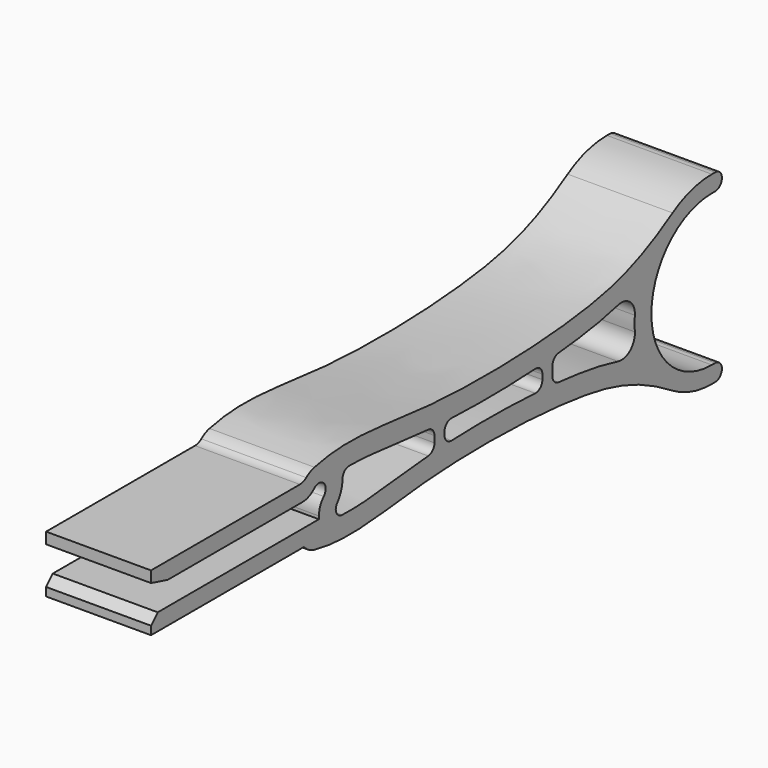
from build123d import *

# Parameters (mm, degrees)
F1_DEPTH    = 25
F2_T        = -5
F3_T1_DEPTH = 25
F3_T3_DEPTH = 35
F4_R        = 5
F5_R        = 3
F6_SIZE2    = 1.3397459622
F6_SIZE     = 5
F7_SIZE     = 2
F8_W        = 3
F8_H        = 15.4217101982
F8_H_2      = 14.9222370414
F9_DEPTH    = 25
F10_R       = 4
F11_R       = 2


# Not quite as in the source:
# - a fillet or chamfer that OpenCascade refuses, or shapes differently, is made with other operations: its cross-section is extruded or revolved along the edge and cut away or added
# - two fillets or chamfers of one size are made in one step


with BuildPart() as f1:
    # F0 (on Right) → F1 (new body)
    with BuildSketch(Plane.YZ):
        with BuildLine():
            Line((0, 0), (-50, 0))
            Line((-50, 0), (-50, -4))
            Line((-50, -4), (-4.472135955, -4))
            ThreePointArc((-4.472135955, -4), (-3.050460985, -5.1666902151), (-1.3421845475, -5.8479518329))
            add(Edge.make_bspline(
                [(-1.3421845475, -5.8479518329), (9.2071972379, -8.2691785501), (31.0373626239, -3.5012878358), (78.4361481231, -4.5602935295), (95.2697355868, -9.5377090854), (105.3076201307, -15.8356715198)],
                knots=[0, 0, 0, 0, 0.3199533187, 0.6955127436, 1, 1, 1, 1], degree=3))
            ThreePointArc((105.3076201307, -15.8356715198), (110.9166116939, -18.3421944631), (117, -19.2))
            Line((117, -19.2), (120, -19.2))
            Line((120, -19.2), (120, -15.2))
            Line((120, -15.2), (117, -15.2))
            ThreePointArc((117, -15.2), (99, 2.8), (117, 20.8))
            Line((117, 20.8), (120, 20.8))
            Line((120, 20.8), (120, 24.8))
            Line((120, 24.8), (117, 24.8))
            ThreePointArc((117, 24.8), (110.9166116939, 23.9421944631), (105.3076201307, 21.4356715198))
            add(Edge.make_bspline(
                [(-1.3421845475, 11.4479518329), (9.2071972379, 13.8691785501), (31.0373626239, 9.1012878358), (78.4361481231, 10.1602935295), (95.2697355868, 15.1377090854), (105.3076201307, 21.4356715198)],
                knots=[0, 0, 0, 0, 0.3199533187, 0.6955127436, 1, 1, 1, 1], degree=3))
            ThreePointArc((-1.3421845475, 11.4479518329), (-3.050460985, 10.7666902151), (-4.472135955, 9.6))
            Line((-4.472135955, 9.6), (-50, 9.6))
            Line((-50, 9.6), (-50, 5.6))
            Line((-50, 5.6), (-2, 5.6))
            ThreePointArc((-2, 5.6), (1.4142135624, 7.0142135624), (0, 3.6))
            Line((0, 3.6), (0, 0))
        make_face()
    extrude(amount=F1_DEPTH)

    # F2
    f2_openings = [f1.faces().sort_by_distance(p)[0] for p in [
        (25, 43.571692, 2.787739),
        (0, 43.571692, 2.787739),
    ]]
    offset(amount=F2_T, openings=f2_openings)

    # F3: fillet of radius 2 on 7 edges, made by hand

    # F3_s2 → F3_t1 (join)
    with BuildSketch(Plane.YZ):
        with BuildLine():
            ThreePointArc((6.9998694988, 5.5572565768), (7.5890521661, 6.9626829324), (8.9973194291, 7.5450425917))
            ThreePointArc((8.9973194291, 7.5450425917), (7.867864466, 7.5318861702), (6.7389684215, 7.4937541059))
            ThreePointArc((6.7389684215, 7.4937541059), (6.9373209901, 6.5346536684), (6.9998694988, 5.5572565768))
        make_face()
        with BuildLine():
            ThreePointArc((5.4442630355, 1.2), (5.1168993976, 0.6172535364), (4.9998334, -0.0408163265))
            Line((4.9998334, -0.0408163265), (4.799840064, -0.0391836735))
            ThreePointArc((4.799840064, -0.0391836735), (4.8, 0), (4.8, 0.7010205144))
            Line((4.8, 0.7010205144), (4.8571428571, 0.8409913569))
            ThreePointArc((4.8571428571, 0.8409913569), (5.0787139257, 1.0782011476), (5.2887126631, 1.3257142857))
            Line((5.2887126631, 1.3257142857), (5.4442630355, 1.2))
        make_face()
        with BuildLine():
            ThreePointArc((5, 0.0967574345), (5.5565984833, -1.2876529316), (6.9165920616, -1.9015025876))
            Line((6.9165920616, -1.9015025876), (6.9082512677, -2.1013285898))
            ThreePointArc((6.9082512677, -2.1013285898), (5.7854909674, -2.0408513189), (4.6642648137, -1.9518448324))
            Line((4.6642648137, -1.9518448324), (4.4954292935, -1.6825918896))
            ThreePointArc((4.4954292935, -1.6825918896), (4.8, 0), (4.8, 0.0967574345))
            Line((4.8, 0.0967574345), (5, 0.0967574345))
        make_face()
    extrude(amount=F3_T1_DEPTH)

    # F3_s4 → F3_t3 (cut)
    with BuildSketch(Plane.YZ.offset(-5)):
        with BuildLine():
            ThreePointArc((118, -15.2), (119.4142135624, -15.7857864376), (120, -17.2))
            Line((120, -17.2), (120, -15.2))
            Line((120, -15.2), (118, -15.2))
        make_face()
        with BuildLine():
            ThreePointArc((120, 22.8), (119.4142135624, 21.3857864376), (118, 20.8))
            Line((118, 20.8), (120, 20.8))
            Line((120, 20.8), (120, 22.8))
        make_face()
        with BuildLine():
            ThreePointArc((118, 24.8), (119.4142135624, 24.2142135624), (120, 22.8))
            Line((120, 22.8), (120, 24.8))
            Line((120, 24.8), (118, 24.8))
        make_face()
        with BuildLine():
            ThreePointArc((120, -17.2), (119.4142135624, -18.6142135624), (118, -19.2))
            Line((118, -19.2), (120, -19.2))
            Line((120, -19.2), (120, -17.2))
        make_face()
    extrude(amount=F3_T3_DEPTH, mode=Mode.SUBTRACT)

    # F4
    f4_edges = [f1.edges().sort_by_distance(p)[0] for p in [
        (12.5, 0, 3.6),
        (12.5, -2, 5.6),
    ]]
    fillet(f4_edges, radius=F4_R)

    # F5
    f5_edges = [f1.edges().sort_by_distance(p)[0] for p in [
        (12.5, -4.472136, 9.6),
    ]]
    fillet(f5_edges, radius=F5_R)

    # F6
    f6_edges = [f1.edges().sort_by_distance(p)[0] for p in [
        (12.5, -50, 5.6),
    ]]
    f6_side = f1.faces().sort_by_distance((12.5, -27.44949, 5.6))[0]
    chamfer(f6_edges, length=F6_SIZE, length2=F6_SIZE2, reference=f6_side)

    # F7
    f7_edges = [f1.edges().sort_by_distance(p)[0] for p in [
        (12.5, -50, 0),
    ]]
    chamfer(f7_edges, length=F7_SIZE)

    # F8 (on face) → F9 (join, through all)
    with BuildSketch(Plane(origin=(0, 0, 0), x_dir=(0, -1, 0), z_dir=(-1, 0, 0))):
        with Locations((-68.0342436071, 2.8)):
            Rectangle(F8_W, F8_H)
        with Locations((-35.897509649, 2.8)):
            Rectangle(F8_W, F8_H_2)
    extrude(amount=-F9_DEPTH)

    # F10
    f10_edges = [f1.edges().sort_by_distance(p)[0] for p in [
        (12.5, 95.426024, -5.172674),
        (12.5, 95.426024, 10.772674),
    ]]
    fillet(f10_edges, radius=F10_R)

    # F11
    f11_edges = [f1.edges().sort_by_distance(p)[0] for p in [
        (12.5, 69.534244, 5.721816),
        (12.5, 69.534244, -0.121816),
        (12.5, 34.39751, 5.429704),
        (12.5, 34.39751, 0.170296),
        (12.5, 37.39751, 5.254407),
        (12.5, 66.534244, 5.499313),
        (12.5, 66.534244, 0.100687),
        (12.5, 37.39751, 0.345593),
    ]]
    fillet(f11_edges, radius=F11_R)


solid = f1.part
